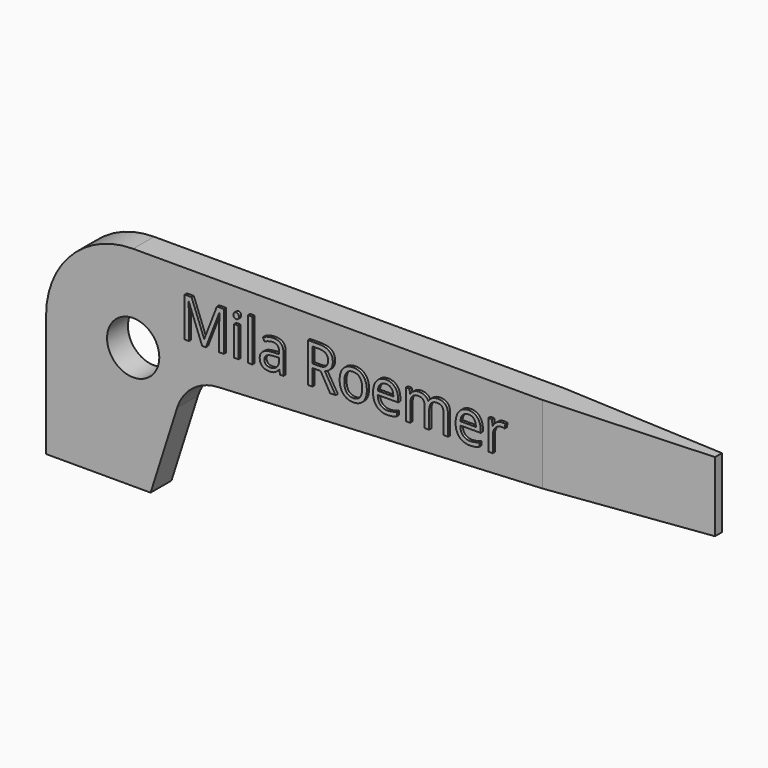
from build123d import *

# Parameters (mm, degrees)
F1_DEPTH     = 2.38125
F2_R         = 2.38125
F3_DEPTH     = 2.38225
F5_DEPTH     = 25.4
F6_TEXT_SIZE = 5.0435062601
F7_DEPTH     = 0.254


# Not quite as in the source:
# - Text() gives the source's letters only with a copy of the font that has no kerning and outlines rounded to 1/6400 em; it was checked with that copy


with BuildPart() as f1:
    # F0 (on Front) → F1 (new body)
    with BuildSketch(Plane.XZ):
        with BuildLine():
            Line((60.325, 19.05), (7.9375, 19.05))
            ThreePointArc((7.9375, 19.05), (2.3248399243, 16.7251600757), (0, 11.1125))
            Line((0, 11.1125), (0, 0))
            Line((0, 0), (9.525, 0))
            Line((9.525, 0), (11.9441518357, 7.6010528185))
            ThreePointArc((11.9441518357, 7.6010528185), (13.3579469744, 9.6182020304), (15.6692569936, 10.4699963909))
            Line((15.6692569936, 10.4699963909), (60.325, 12.7))
            Line((60.325, 12.7), (60.325, 19.05))
        make_face()
    extrude(amount=F1_DEPTH)

    # F2 (on face) → F3 (cut, through all)
    with BuildSketch(Plane.XZ.offset(2.38125)):
        with Locations((7.9375, 11.1125)):
            Circle(F2_R)
    extrude(amount=-F3_DEPTH, mode=Mode.SUBTRACT)

    # F4 (on face) → F5 (cut)
    with BuildSketch(Plane.XY.offset(19.05)):
        Polygon((60.325, 0), (45.24375, 0), (60.325, -0.79375), align=None)
        Polygon((60.325, -2.38125), (60.325, -1.5875), (45.24375, -2.38125), align=None)
    extrude(amount=-F5_DEPTH, mode=Mode.SUBTRACT)

    # F6 (on face) → F7 (join)
    with BuildSketch(Plane.XZ.offset(2.38125)):
        with Locations((12.3373987153, 13.4692480788)):
            Text('Mila Roemer', F6_TEXT_SIZE, font='Open Sans', text_align=(TextAlign.LEFT, TextAlign.BOTTOM))
    extrude(amount=F7_DEPTH)


solid = f1.part
